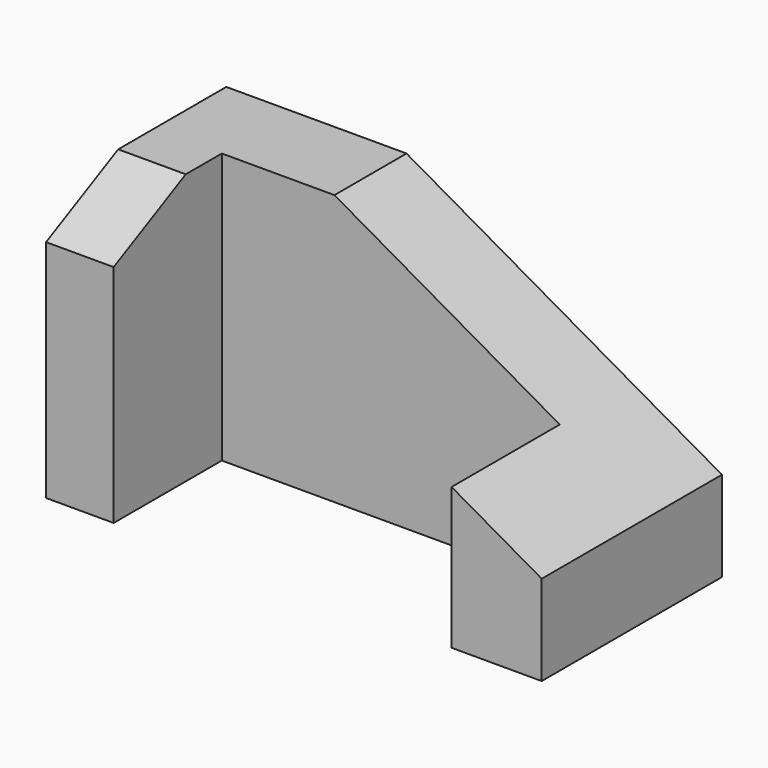
from build123d import *

# Parameters (mm, degrees)
F2_DEPTH = 60
F4_DEPTH = 15
F6_DEPTH = 50


# Not quite as in the source:
# - a feature names something its author has since deleted; it is built from what else it names


with BuildPart() as f2:
    # F1 (on Top) → F2 (new body)
    with BuildSketch(Plane.XY):
        Polygon((0, 50), (0, 0), (15, 0), (15, 30), (90, 30), (90, 0), (110, 0), (110, 50), align=None)
    extrude(amount=F2_DEPTH)

    # F3 (on face) → F4 (cut)
    with BuildSketch(Plane(origin=(0, 0, 0), x_dir=(0, -1, 0), z_dir=(-1, 0, 0))):
        Polygon((0, 50), (0, 60), (-20, 60), align=None)
    extrude(amount=-F4_DEPTH, mode=Mode.SUBTRACT)

    # F5 (on face) → F6 (cut)
    with BuildSketch(Plane(origin=(0, 50, 0), x_dir=(-1, 0, 0), z_dir=(0, 1, 0))):
        Polygon((-110, 20), (-40, 60), (-110, 60), align=None)
    extrude(amount=-F6_DEPTH, mode=Mode.SUBTRACT)


solid = f2.part
